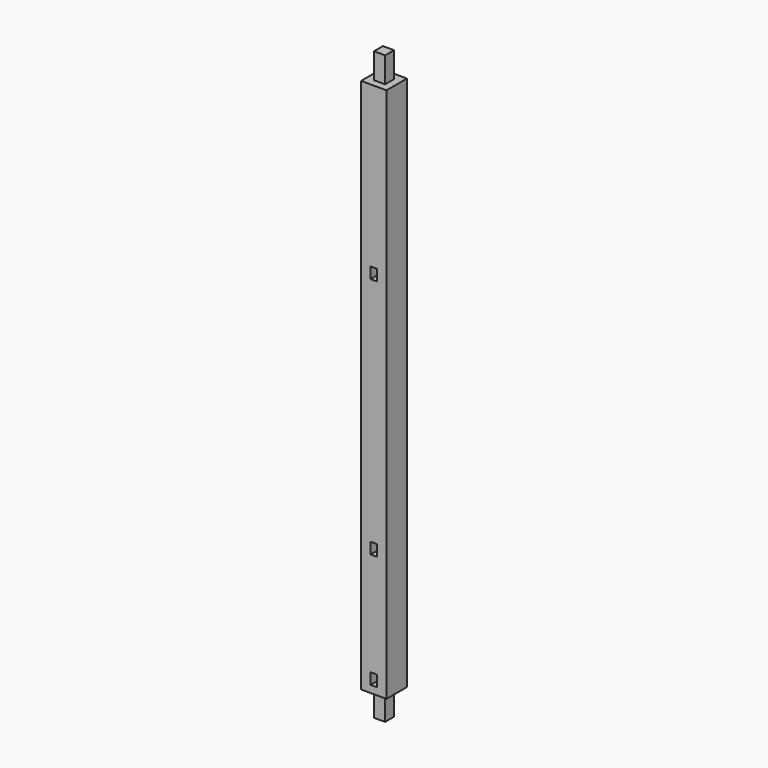
from build123d import *

# Parameters (mm, degrees)
F0_W     = 101.6
F0_H     = 101.6
F1_DEPTH = 1168.4
F2_W     = 101.6
F2_H     = 101.6
F2_W_2   = 44.45
F2_H_2   = 44.45
F3_DEPTH = 101.6
F4_W     = 25.4
F4_H     = 44.45
F5_DEPTH = 101.601
F6_W     = 25.4
F6_H     = 44.45
F7_DEPTH = 101.601
F8_W     = 25.4
F8_H     = 44.45
F9_DEPTH = 101.601


# Not quite as in the source:
# - a pattern or mirror of a feature is missing from the dataset's text; its kind, count and spacing are read off the source's solid


with BuildPart() as f1:
    # F0 (on Top) → F1 (new body, symmetric)
    with BuildSketch(Plane.XY):
        Rectangle(F0_W, F0_H)
    extrude(amount=F1_DEPTH, both=True)

    # F2 (on face) → F3 (cut)
    with BuildSketch(Plane.XY.offset(1168.4)):
        Rectangle(F2_W, F2_H)
        Rectangle(F2_W_2, F2_H_2, mode=Mode.SUBTRACT)
    f3 = extrude(amount=-F3_DEPTH, mode=Mode.SUBTRACT)

    # F3_copies: F3 across plane
    add(f3.mirror(Plane(origin=(0, 0, 0), x_dir=(-1, 0, 0), z_dir=(0, 0, -1))), mode=Mode.SUBTRACT)

    # F4 (on face) → F5 (cut, through all)
    with BuildSketch(Plane.XZ.offset(50.8)):
        with Locations((0, 406.4)):
            Rectangle(F4_W, F4_H)
    extrude(amount=-F5_DEPTH, mode=Mode.SUBTRACT)

    # F6 (on face) → F7 (cut, through all)
    with BuildSketch(Plane(origin=(0, 50.8, 0), x_dir=(-1, 0, 0), z_dir=(0, 1, 0))):
        with Locations((0, -558.8)):
            Rectangle(F6_W, F6_H)
    extrude(amount=-F7_DEPTH, mode=Mode.SUBTRACT)

    # F8 (on face) → F9 (cut, through all)
    with BuildSketch(Plane(origin=(0, 50.8, 0), x_dir=(-1, 0, 0), z_dir=(0, 1, 0))):
        with Locations((0, -1016)):
            Rectangle(F8_W, F8_H)
    extrude(amount=-F9_DEPTH, mode=Mode.SUBTRACT)


solid = f1.part
